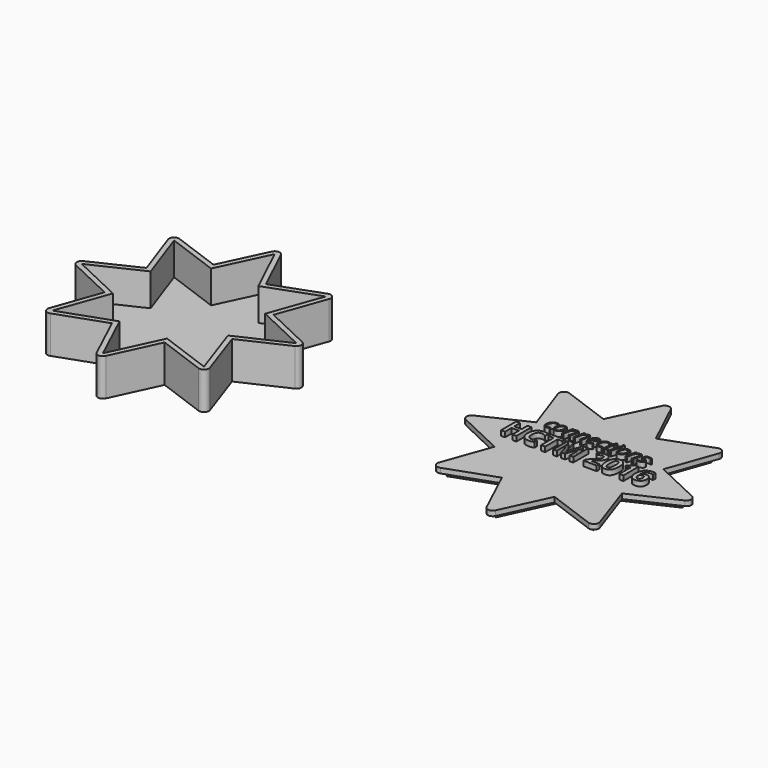
from build123d import *

# Parameters (mm, degrees)
F1_DEPTH       = 5.08
F2_DEPTH       = 2.54
F3_DEPTH       = 19.05
F4_T           = -2.54
F5_R           = 2.54
F5_2_R         = 2.54
F6_TEXT_SIZE   = 9.9312410586
F6_TEXT_SIZE_2 = 13.3956265118
F7_DEPTH       = 2.54


# Not quite as in the source:
# - Text() gives the source's letters only with a copy of the font that has no kerning and outlines rounded to 1/6400 em; it was checked with that copy


with BuildPart() as f1:
    # F0 (on Top) → F1 (new body)
    with BuildSketch(Plane.XY):
        Polygon((181.1209609165, 74.4860608765), (169.4359795465, 49.7724338682), (143.6053853116, 59.2264335926), (152.7358891383, 33.3308782948), (128.0662802247, 21.6169280816), (152.8696337201, 9.8854726312), (143.6190827071, -15.9023723964), (169.4573394718, -6.7556298984), (181.1017875648, -31.5708283169), (192.7346669247, -6.499488186), (218.5418361777, -15.9511590399), (209.5121154407, 10.1529431579), (234.1575086395, 21.6335851606), (209.3444118192, 33.3712377869), (218.5740669155, 59.139311767), (192.8423919959, 49.7426088385), align=None)
    extrude(amount=-F1_DEPTH)

    # F0 (on Top) → F2 (join)
    with BuildSketch(Plane.XY):
        Polygon((194.4924095296, 53.7666657474), (181.1181889498, 81.9990874734), (167.7848320105, 53.7991614547), (138.3071155869, 64.5880082157), (148.7422274076, 34.9923779722), (120.5615276122, 21.6112451162), (148.8601365709, 8.2266086247), (138.3071118616, -21.1921541486), (167.7848301479, -10.7570423279), (181.1181889498, -39.1714370344), (194.4056391367, -10.5341433082), (223.7916202866, -21.2965256069), (213.497167977, 8.463800652), (241.7206713581, 21.6112451162), (213.3526006364, 35.0305519532), (223.9115932607, 64.5099745598), align=None)
        Polygon((143.6053853116, 59.2264335926), (169.4359795465, 49.7724338682), (181.1209609165, 74.4860608765), (192.8423919959, 49.7426088385), (218.5740669155, 59.139311767), (209.3444118192, 33.3712377869), (234.1575086395, 21.6335851606), (209.5121154407, 10.1529431579), (218.5418361777, -15.9511590399), (192.7346669247, -6.499488186), (181.1017875648, -31.5708283169), (169.4573394718, -6.7556298984), (143.6190827071, -15.9023723964), (152.8696337201, 9.8854726312), (128.0662802247, 21.6169280816), (152.7358891383, 33.3308782948), align=None, mode=Mode.SUBTRACT)
    extrude(amount=-F2_DEPTH)

    # F5
    f5_edges = [f1.edges().sort_by_distance(p)[0] for p in [
        (223.79162, -21.296526, -1.27),
        (181.118189, -39.171437, -1.27),
        (241.720671, 21.611245, -1.27),
        (223.911593, 64.509975, -1.27),
        (181.118189, 81.999087, -1.27),
        (138.307112, -21.192154, -1.27),
        (120.561528, 21.611245, -1.27),
        (138.307116, 64.588008, -1.27),
    ]]
    fillet(f5_edges, radius=F5_R)

    # F6 (on face) → F7 (join)
    with BuildSketch(Plane.XY):
        with Locations((155.165836215, 30.4172448814)):
            Text('connections', F6_TEXT_SIZE, font='Open Sans', font_style=FontStyle.ITALIC, text_align=(TextAlign.LEFT, TextAlign.BOTTOM))
        with Locations((143.8581049442, 17.1140013263)):
            Text('HCTM 2016', F6_TEXT_SIZE_2, font='Open Sans', font_style=FontStyle.BOLD, text_align=(TextAlign.LEFT, TextAlign.BOTTOM))
    extrude(amount=F7_DEPTH)


with BuildPart() as f3:
    # F0 (on Top) → F3 (new body)
    with BuildSketch(Plane.XY):
        Polygon((13.3742205799, 32.1554206312), (0, 60.3878423572), (-13.3333569393, 32.1879163384), (-42.8110733628, 42.9767630994), (-32.3759615421, 13.381132856), (-60.5566613376, 0), (-32.2580523789, -13.3846364915), (-42.8110770881, -42.8033992648), (-13.3333588019, -32.3682874441), (0, -60.7826821506), (13.2874501869, -32.1453884244), (42.6734313369, -42.9077707231), (32.3789790273, -13.1474444643), (60.6024824083, 0), (32.2344116867, 13.419306837), (42.7934043109, 42.8987294436), align=None)
    extrude(amount=F3_DEPTH)

    # F4
    f4_openings = [f3.faces().sort_by_distance(p)[0] for p in [
        (-0.034563, -0.043411, 19.05),
    ]]
    offset(amount=F4_T, openings=f4_openings, kind=Kind.INTERSECTION)

    # F5#2
    f5_2_edges = [f3.edges().sort_by_distance(p)[0] for p in [
        (60.602482, 0, 9.525),
        (42.673431, -42.907771, 9.525),
        (0, -60.782682, 9.525),
        (-42.811077, -42.803399, 9.525),
        (-60.556661, 0, 9.525),
        (-42.811073, 42.976763, 9.525),
        (42.793404, 42.898729, 9.525),
        (0, 60.387842, 9.525),
    ]]
    fillet(f5_2_edges, radius=F5_2_R)


solid = Compound([f1.part, f3.part])
